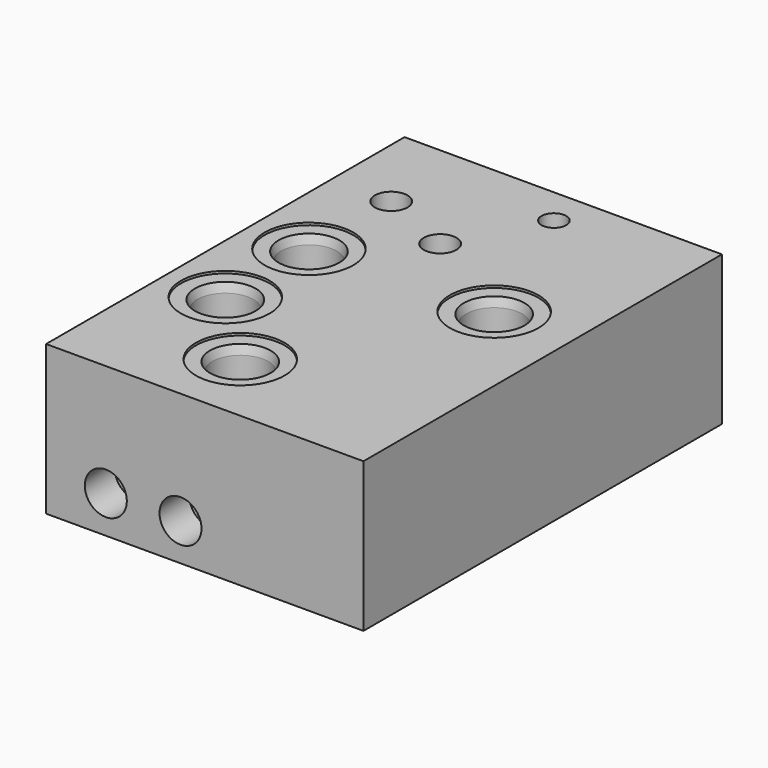
from build123d import *

# Parameters (mm, degrees)
F0_W           = 107.95
F0_H           = 152.4
F1_DEPTH       = 25.4
F18_R          = 7.14375
F19_DEPTH      = 12.7
F20_R          = 4.7625
F21_DEPTH      = 101.6
F22_R          = 7.14375
F23_DEPTH      = 12.7
F24_R          = 4.7625
F25_DEPTH      = 101.6
F26_R          = 5.9436
F27_DEPTH      = 4.7752
F28_R          = 1.5875
F29_DEPTH      = 3.175
F31_DEPTH      = 22.86
F32_R          = 7.14375
F32_R_2        = 4.7625
F33_DEPTH      = 12.7
F34_END_RADIUS = 8.7376
F34_REACH      = 165.8713841816
F35_R          = 7.14375
F35_R_2        = 4.7625
F36_DEPTH      = 12.7
F37_R          = 5.9436
F38_DEPTH      = 4.7752
F39_DEPTH      = 31.75
F40_R          = 5.5626
F41_DEPTH      = 15.875


# Not quite as in the source:
# - a feature names something its author has since deleted; it is built from what else it names


with BuildPart() as f1:
    # F0 (on Top) → F1 (new body, symmetric)
    with BuildSketch(Plane.XY):
        Rectangle(F0_W, F0_H)
    extrude(amount=F1_DEPTH, both=True)

    # F3 (on offset) → F4 (revolve, cut)
    with BuildSketch(Plane.XZ.offset(50.8)):
        Polygon((6.8326, 25.4), (-8.255, 25.4), (-8.255, -3.9624), (-1.905, -3.9624), (-1.905, 6.35), (0.4826, 6.35), (0.4826, 12.7), (1.27, 12.7), (1.27, 21.6265861489), (2.0701, 24.6126), (6.8326, 24.6126), align=None)
    revolve(axis=Axis((-8.255, -50.8, 4.1184453023), (0, 0, -1)), mode=Mode.SUBTRACT)

    # F6 (on offset) → F7 (revolve, cut)
    with BuildSketch(Plane.XZ.offset(25.4)):
        Polygon((-18.5674, 25.4), (-33.655, 25.4), (-33.655, -3.9624), (-27.305, -3.9624), (-27.305, 6.35), (-24.9174, 6.35), (-24.9174, 12.7), (-24.13, 12.7), (-24.13, 21.6265861489), (-23.3299, 24.6126), (-18.5674, 24.6126), align=None)
    revolve(axis=Axis((-33.655, -25.4, 7.4702984761), (0, 0, -1)), mode=Mode.SUBTRACT)

    # F9 (on offset) → F10 (revolve, cut)
    with BuildSketch(Plane.XZ.offset(-63.5)):
        Polygon((11.2014, -3.8165312859), (11.2014, 25.4), (6.985, 25.4), (6.985, -6.35), align=None)
    revolve(axis=Axis((6.985, 63.5, 7.0877279262), (0, 0, -1)), mode=Mode.SUBTRACT)

    # F12 (on offset) → F13 (revolve, cut)
    with BuildSketch(Plane.XZ.offset(-12.7)):
        Polygon((42.3926, 25.4), (27.305, 25.4), (27.305, -3.9624), (33.655, -3.9624), (33.655, 6.35), (36.0426, 6.35), (36.0426, 12.7), (36.83, 12.7), (36.83, 21.6265861489), (37.6301, 24.6126), (42.3926, 24.6126), align=None)
    revolve(axis=Axis((27.305, 12.7, 8.8350928114), (0, 0, -1)), mode=Mode.SUBTRACT)

    # F15 (on offset) → F16 (revolve, cut)
    with BuildSketch(Plane.XZ.offset(-10.16)):
        Polygon((-18.5674, 25.4), (-33.655, 25.4), (-33.655, -3.9624), (-27.305, -3.9624), (-27.305, 6.35), (-24.9174, 6.35), (-24.9174, 12.7), (-24.13, 12.7), (-24.13, 21.6265861489), (-23.3299, 24.6126), (-18.5674, 24.6126), align=None)
    revolve(axis=Axis((-33.655, 10.16, 10.2464657762), (0, 0, -1)), mode=Mode.SUBTRACT)

    # F18 (on face) → F19 (cut)
    with BuildSketch(Plane.XZ.offset(76.2)):
        with Locations((-33.655, -12.7)):
            Circle(F18_R)
    extrude(amount=-F19_DEPTH, mode=Mode.SUBTRACT)

    # F20 (on face) → F21 (cut)
    with BuildSketch(Plane.XZ.offset(76.2)):
        with Locations((-33.655, -12.7)):
            Circle(F20_R)
    extrude(amount=-F21_DEPTH, mode=Mode.SUBTRACT)

    # F22 (on face) → F23 (cut)
    with BuildSketch(Plane(origin=(0, 76.2, 0), x_dir=(-1, 0, 0), z_dir=(0, 1, 0))):
        with Locations((33.655, 10.9728)):
            Circle(F22_R)
    extrude(amount=-F23_DEPTH, mode=Mode.SUBTRACT)

    # F24 (on face) → F25 (cut)
    with BuildSketch(Plane(origin=(0, 76.2, 0), x_dir=(-1, 0, 0), z_dir=(0, 1, 0))):
        with Locations((33.655, 10.9728)):
            Circle(F24_R)
    extrude(amount=-F25_DEPTH, mode=Mode.SUBTRACT)

    # F26 (on face) → F27 (cut)
    with BuildSketch(Plane.XY.offset(-3.9624)):
        with Locations((-33.655, 10.16)):
            Circle(F26_R)
    extrude(amount=-F27_DEPTH, mode=Mode.SUBTRACT)

    # F28 (on face) → F29 (cut)
    with BuildSketch(Plane.XY.offset(-3.9624)):
        with Locations((-33.655, -20.6375)):
            Circle(F28_R)
    extrude(amount=-F29_DEPTH, mode=Mode.SUBTRACT)

    # F30 (on face) → F31 (cut)
    with BuildSketch(Plane(origin=(-53.975, 0, 0), x_dir=(0, -1, 0), z_dir=(-1, 0, 0))):
        with BuildLine():
            ThreePointArc((21.7122081883, -7.1374), (22.0911601217, -6.606987853), (22.225, -5.969))
            ThreePointArc((22.225, -5.969), (19.999512147, -4.5153398783), (19.5627918117, -7.1374))
            Line((19.5627918117, -7.1374), (21.7122081883, -7.1374))
        make_face()
        with BuildLine():
            Line((21.7122081883, -7.1374), (19.5627918117, -7.1374))
            ThreePointArc((19.5627918117, -7.1374), (20.6375, -7.5565), (21.7122081883, -7.1374))
        make_face()
    extrude(amount=-F31_DEPTH, mode=Mode.SUBTRACT)

    # F32 (on face) → F33 (cut, through all)
    with BuildSketch(Plane(origin=(0, 76.2, 0), x_dir=(-1, 0, 0), z_dir=(0, 1, 0))):
        with Locations((8.255, 10.9728)):
            Circle(F32_R)
        with Locations((8.255, 10.9728)):
            Circle(F32_R_2, mode=Mode.SUBTRACT)
        with Locations((8.255, 10.9728)):
            Circle(F32_R_2)
    extrude(amount=-F33_DEPTH, mode=Mode.SUBTRACT)

    f34_end = (Plane(origin=(-8.255, -50.8, 9.525), x_dir=(1, 0, 0), z_dir=(0, 0, 1)) * Cylinder(F34_END_RADIUS, 718.8324349781, mode=Mode.PRIVATE)).faces().sort_by_distance((-16.9926, -50.8, 9.525))[0]
    # F32 (on face) → F34 (cut, up to the whole of a round face its end follows)
    with BuildSketch(Plane(origin=(0, 76.2, 0), x_dir=(-1, 0, 0), z_dir=(0, 1, 0))):
        with Locations((8.255, 10.9728)):
            Circle(F32_R_2)
    f34_long = extrude(amount=-F34_REACH, mode=Mode.PRIVATE)
    add(split(f34_long, bisect_by=f34_end, keep=Keep.ALL, mode=Mode.PRIVATE).solids().sort_by_distance((-8.255, 76.2, 10.9728))[0], mode=Mode.SUBTRACT)

    # F35 (on face) → F36 (cut, through all)
    with BuildSketch(Plane.XZ.offset(76.2)):
        with Locations((-8.255, -12.7)):
            Circle(F35_R)
        with Locations((-8.255, -12.7)):
            Circle(F35_R_2, mode=Mode.SUBTRACT)
    extrude(amount=-F36_DEPTH, mode=Mode.SUBTRACT)

    # F37 (on face) → F38 (cut, through all)
    with BuildSketch(Plane.XY.offset(-3.9624)):
        with Locations((-8.255, -50.8)):
            Circle(F37_R)
    extrude(amount=-F38_DEPTH, mode=Mode.SUBTRACT)

    # F39 (cut): a face of the model
    f39_faces = [f1.faces().sort_by_distance(p)[0] for p in [
        (-8.255, -76.2, -12.7),
    ]]
    extrude(f39_faces, amount=-F39_DEPTH, mode=Mode.SUBTRACT)

    # F40 (on face) → F41 (cut)
    with BuildSketch(Plane.XY.offset(25.4)):
        with Locations((-8.255, 34.1804362833)):
            Circle(F40_R)
        with Locations((-33.655, 45.1278984547)):
            Circle(F40_R)
    extrude(amount=-F41_DEPTH, mode=Mode.SUBTRACT)


solid = f1.part
